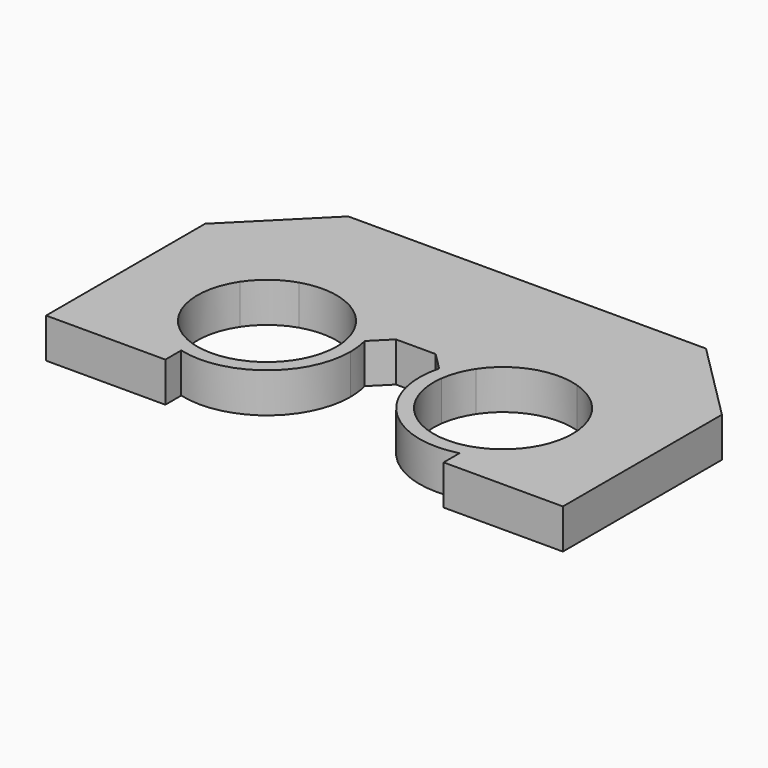
from build123d import *

# Parameters (mm, degrees)
F1_DEPTH = 10


with BuildPart() as f1:
    # F0 (on Top) → F1 (new body)
    with BuildSketch(Plane.XY):
        with BuildLine():
            Line((45, 0), (0, 0))
            Line((0, 0), (0, -35))
            Line((0, -35), (5, -35))
            Line((5, -35), (11.0542490694, -35))
            ThreePointArc((11.0542490694, -35), (21.1660409917, -25.4925456214), (35, -24.3693346885))
            Line((35, -24.3693346885), (35, -20))
            Line((35, -20), (45, -20))
            Line((45, -20), (45, 0))
        make_face()
        with BuildLine():
            Line((0, -35), (0, 0))
            Line((0, 0), (-45, 0))
            Line((-45, 0), (-45, -20))
            Line((-45, -20), (-35, -20))
            Line((-35, -20), (-35, -24.3693346885))
            ThreePointArc((-35, -24.3693346885), (-21.1660409917, -25.4925456214), (-11.0542490694, -35))
            Line((-11.0542490694, -35), (-5, -35))
            Line((-5, -35), (0, -35))
        make_face()
        Polygon((65, -20), (45, 0), (45, -20), align=None)
        Polygon((-45, -20), (-45, 0), (-65, -20), align=None)
        with BuildLine():
            Line((65, -20), (45, -20))
            Line((45, -20), (45, -30.3156087011))
            ThreePointArc((45, -30.3156087011), (49.2135509862, -36.9586799562), (50.6869892627, -44.6861237288))
            ThreePointArc((50.6869892627, -44.6861237288), (46.3088607801, -57.5201950726), (35, -65.002912769))
            Line((35, -65.002912769), (35, -70))
            Line((35, -70), (65, -70))
            Line((65, -70), (65, -20))
        make_face()
        with BuildLine():
            Line((45, -30.3156087011), (45, -20))
            Line((45, -20), (35, -20))
            Line((35, -20), (35, -24.3693346885))
            ThreePointArc((35, -24.3693346885), (40.420009999, -26.6361302142), (45, -30.3156087011))
        make_face()
        with BuildLine():
            Line((11.0542490694, -35), (5, -35))
            Line((5, -35), (9.3708041453, -39.3708041453))
            ThreePointArc((9.3708041453, -39.3708041453), (10.0902885727, -37.1383212628), (11.0542490694, -35))
        make_face()
        with BuildLine():
            Line((-9.3708041453, -39.3708041453), (-5, -35))
            Line((-5, -35), (-11.0542490694, -35))
            ThreePointArc((-11.0542490694, -35), (-10.0902885727, -37.1383212628), (-9.3708041453, -39.3708041453))
        make_face()
        with BuildLine():
            Line((-35, -20), (-45, -20))
            Line((-45, -20), (-45, -30.3156087011))
            ThreePointArc((-45, -30.3156087011), (-40.420009999, -26.6361302142), (-35, -24.3693346885))
            Line((-35, -24.3693346885), (-35, -20))
        make_face()
        with BuildLine():
            Line((-45, -30.3156087011), (-45, -20))
            Line((-45, -20), (-65, -20))
            Line((-65, -20), (-65, -70))
            Line((-65, -70), (-35, -70))
            Line((-35, -70), (-35, -65.002912769))
            ThreePointArc((-35, -65.002912769), (-49.8652066354, -50.5033003341), (-45, -30.3156087011))
        make_face()
        with BuildLine():
            ThreePointArc((50.6869892627, -44.6861237288), (49.2135509862, -36.9586799562), (45, -30.3156087011))
            Line((45, -30.3156087011), (45, -35))
            Line((45, -35), (44.2619337604, -35))
            ThreePointArc((44.2619337604, -35), (46.439773042, -39.6270491449), (47.1869892627, -44.6861237288))
            ThreePointArc((47.1869892627, -44.6861237288), (43.815465612, -55.0126021241), (35, -61.3601129606))
            Line((35, -61.3601129606), (35, -65))
            Line((35, -65), (35, -65.002912769))
            ThreePointArc((35, -65.002912769), (46.3088607801, -57.5201950726), (50.6869892627, -44.6861237288))
        make_face()
        with BuildLine():
            Line((45, -35), (45, -30.3156087011))
            ThreePointArc((45, -30.3156087011), (40.420009999, -26.6361302142), (35, -24.3693346885))
            Line((35, -24.3693346885), (35, -28.0121344969))
            ThreePointArc((35, -28.0121344969), (40.2269255495, -30.7161651365), (44.2619337604, -35))
            Line((44.2619337604, -35), (45, -35))
        make_face()
        with BuildLine():
            ThreePointArc((35, -24.3693346885), (21.1660409917, -25.4925456214), (11.0542490694, -35))
            Line((11.0542490694, -35), (15.112044765, -35))
            ThreePointArc((15.112044765, -35), (23.8858324541, -28.1756246545), (35, -28.0121344969))
            Line((35, -28.0121344969), (35, -24.3693346885))
        make_face()
        with BuildLine():
            Line((15.112044765, -35), (11.0542490694, -35))
            ThreePointArc((11.0542490694, -35), (10.0902885727, -37.1383212628), (9.3708041453, -39.3708041453))
            Line((9.3708041453, -39.3708041453), (12.344376437, -42.344376437))
            ThreePointArc((12.344376437, -42.344376437), (13.311166148, -38.5150284196), (15.112044765, -35))
        make_face()
        with BuildLine():
            Line((12.344376437, -42.344376437), (9.3708041453, -39.3708041453))
            ThreePointArc((9.3708041453, -39.3708041453), (14.8369031184, -59.5345223463), (35, -65.002912769))
            Line((35, -65.002912769), (35, -65))
            Line((35, -65), (32.0287365544, -62.0287365544))
            ThreePointArc((32.0287365544, -62.0287365544), (17.3126205919, -57.0604923995), (12.344376437, -42.344376437))
        make_face()
        with BuildLine():
            Line((-12.344376437, -42.344376437), (-9.3708041453, -39.3708041453))
            ThreePointArc((-9.3708041453, -39.3708041453), (-10.0902885727, -37.1383212628), (-11.0542490694, -35))
            Line((-11.0542490694, -35), (-15.112044765, -35))
            ThreePointArc((-15.112044765, -35), (-13.311166148, -38.5150284196), (-12.344376437, -42.344376437))
        make_face()
        with BuildLine():
            ThreePointArc((-8.6869892627, -44.6861237288), (-8.8586445437, -42.006561028), (-9.3708041453, -39.3708041453))
            Line((-9.3708041453, -39.3708041453), (-12.344376437, -42.344376437))
            ThreePointArc((-12.344376437, -42.344376437), (-12.2263803894, -43.5126085924), (-12.1869892627, -44.6861237288))
            ThreePointArc((-12.1869892627, -44.6861237288), (-18.1702748355, -57.8624391774), (-32.0287365544, -62.0287365544))
            Line((-32.0287365544, -62.0287365544), (-35, -65))
            Line((-35, -65), (-35, -65.002912769))
            ThreePointArc((-35, -65.002912769), (-16.8529179189, -61.3079952462), (-8.6869892627, -44.6861237288))
        make_face()
        with BuildLine():
            Line((-15.112044765, -35), (-11.0542490694, -35))
            ThreePointArc((-11.0542490694, -35), (-21.1660409917, -25.4925456214), (-35, -24.3693346885))
            Line((-35, -24.3693346885), (-35, -28.0121344969))
            ThreePointArc((-35, -28.0121344969), (-23.8858324541, -28.1756246545), (-15.112044765, -35))
        make_face()
        with BuildLine():
            ThreePointArc((-35, -24.3693346885), (-40.420009999, -26.6361302142), (-45, -30.3156087011))
            Line((-45, -30.3156087011), (-45, -35))
            Line((-45, -35), (-44.2619337604, -35))
            ThreePointArc((-44.2619337604, -35), (-40.2269255495, -30.7161651365), (-35, -28.0121344969))
            Line((-35, -28.0121344969), (-35, -24.3693346885))
        make_face()
        with BuildLine():
            Line((-45, -35), (-45, -30.3156087011))
            ThreePointArc((-45, -30.3156087011), (-49.8652066354, -50.5033003341), (-35, -65.002912769))
            Line((-35, -65.002912769), (-35, -65))
            Line((-35, -65), (-35, -61.3601129606))
            ThreePointArc((-35, -61.3601129606), (-46.197488337, -50.4872805374), (-44.2619337604, -35))
            Line((-44.2619337604, -35), (-45, -35))
        make_face()
        with BuildLine():
            ThreePointArc((35, -61.3601129606), (33.5289411752, -61.7591845411), (32.0287365544, -62.0287365544))
            Line((32.0287365544, -62.0287365544), (35, -65))
            Line((35, -65), (35, -61.3601129606))
        make_face()
        with BuildLine():
            Line((-35, -65), (-32.0287365544, -62.0287365544))
            ThreePointArc((-32.0287365544, -62.0287365544), (-33.5289411752, -61.7591845411), (-35, -61.3601129606))
            Line((-35, -61.3601129606), (-35, -65))
        make_face()
    extrude(amount=F1_DEPTH)


solid = f1.part
